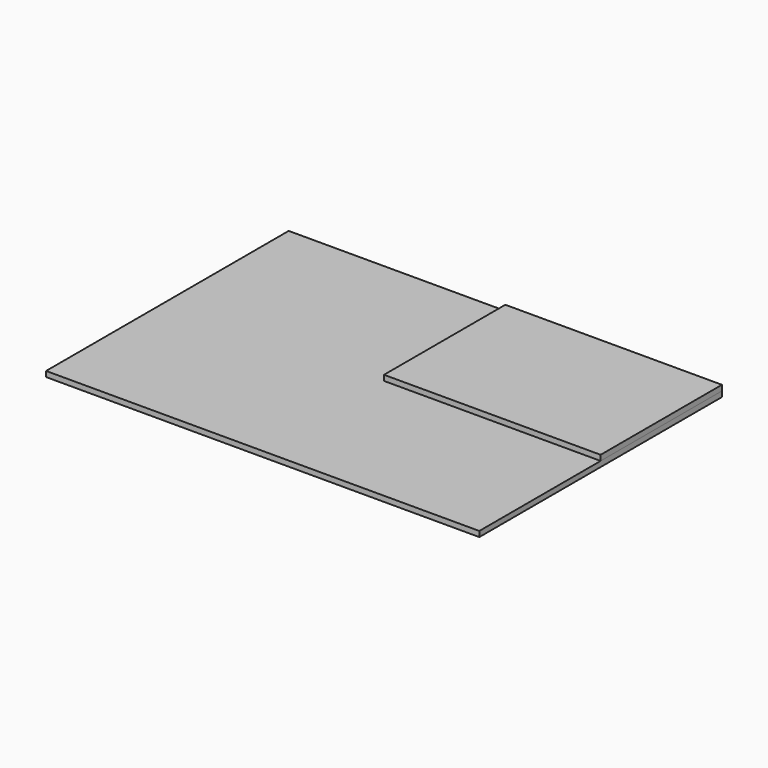
from build123d import *

# Parameters (mm, degrees)
F0_W     = 200
F0_H     = 140
F1_DEPTH = 2.5
F2_W     = 100
F2_H     = 70
F3_DEPTH = 2.5


# Not quite as in the source:
# - a feature names something its author has since deleted; it is built from what else it names


with BuildPart() as f1:
    # F0 (on Top) → F1 (new body)
    with BuildSketch(Plane.XY):
        Rectangle(F0_W, F0_H)
    extrude(amount=F1_DEPTH)


with BuildPart() as f3:
    # F2 (on face) → F3 (new body)
    with BuildSketch(Plane.XY.offset(2.5)):
        with Locations((50, 35)):
            Rectangle(F2_W, F2_H)
    extrude(amount=F3_DEPTH)


solid = Compound([f1.part, f3.part])
